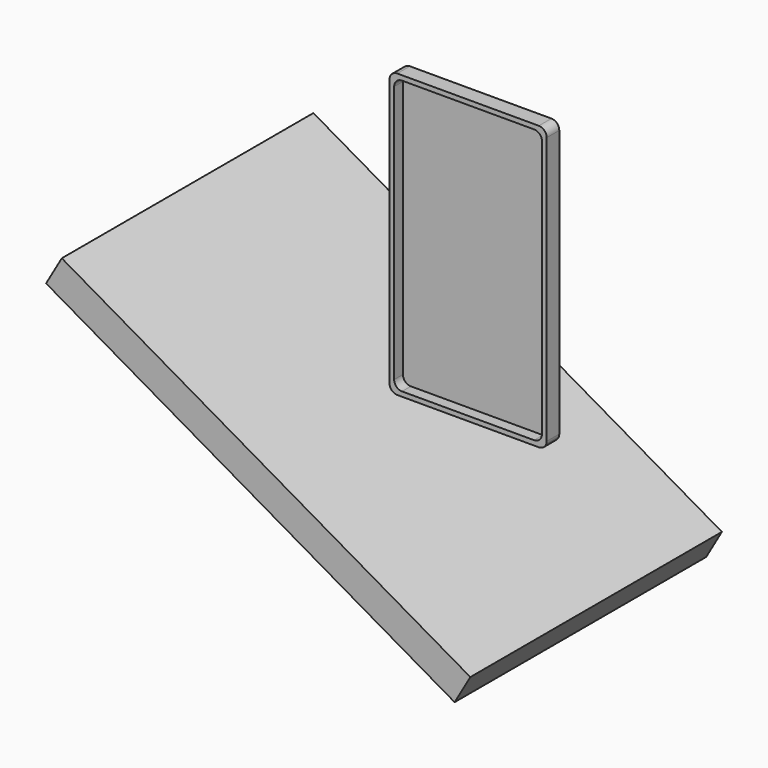
from build123d import *

# Parameters (mm, degrees)
F0_W     = 100
F0_H     = 180
F1_DEPTH = 10
F2_W     = 94
F2_H     = 174
F3_DEPTH = 7
F6_W     = 300
F6_H     = 200
F7_DEPTH = 20
F8_R     = 5


with BuildPart() as f1:
    # F0 (on Front) → F1 (new body)
    with BuildSketch(Plane.XZ):
        Rectangle(F0_W, F0_H)
    extrude(amount=F1_DEPTH)

    # F2 (on face) → F3 (cut)
    with BuildSketch(Plane.XZ.offset(10)):
        Rectangle(F2_W, F2_H)
    extrude(amount=-F3_DEPTH, mode=Mode.SUBTRACT)

    # F8
    f8_edges = [f1.edges().sort_by_distance(p)[0] for p in [
        (-47, -6.5, -87),
        (50, -5, 90),
        (-50, -5, 90),
        (-47, -6.5, 87),
        (47, -6.5, -87),
        (-50, -5, -90),
        (47, -6.5, 87),
        (50, -5, -90),
    ]]
    fillet(f8_edges, radius=F8_R)


with BuildPart() as f7:
    # F6 (on face) → F7 (new body)
    with BuildSketch(Plane(origin=(-66.4711431703, 0, -115.1313972081), x_dir=(0.8660254038, 0, -0.5), z_dir=(0.5, 0, 0.8660254038))):
        Rectangle(F6_W, F6_H)
    extrude(amount=F7_DEPTH)


solid = Compound([f1.part, f7.part])
